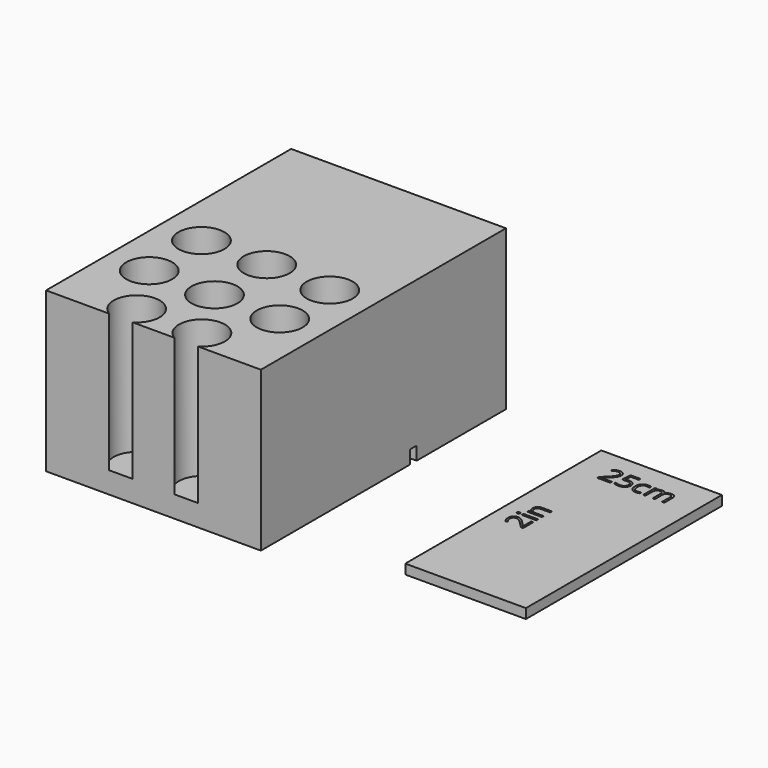
from build123d import *

# Parameters (mm, degrees)
F0_W     = 44.5262
F0_H     = 63.5
F1_DEPTH = 33.02
F2_W     = 44.5262
F2_H     = 1.778
F3_DEPTH = 2.7686
F4_R     = 4.7625
F5_DEPTH = 28.575
F6_W     = 25
F6_H     = 50.8
F6_W_2   = 3.0738876539
F6_H_2   = 0.4657949467
F7_DEPTH = 2


# Not quite as in the source:
# - a length typed as a fraction of an inch, garbled in the dataset ("3 / 203.2 mm" for 3/8 in), is restored


with BuildPart() as f1:
    # F0 (on Top) → F1 (new body)
    with BuildSketch(Plane.XY):
        Rectangle(F0_W, F0_H)
    extrude(amount=F1_DEPTH)

    # F2 (on face) → F3 (cut)
    with BuildSketch(Plane(origin=(0, 0, 0), x_dir=(1, 0, 0), z_dir=(0, 0, -1))):
        with Locations((0, -7.7216)):
            Rectangle(F2_W, F2_H)
    extrude(amount=-F3_DEPTH, mode=Mode.SUBTRACT)

    # F4 (on face) → F5 (cut)
    with BuildSketch(Plane.XY.offset(33.02)):
        with Locations((0, -15.9420263954)):
            Circle(F4_R)
        with Locations((-13.525, -15.9420263954)):
            Circle(F4_R)
        with Locations((13.525, -15.9420263954)):
            Circle(F4_R)
        with Locations((-6.7625, -27.6550199815)):
            Circle(F4_R)
        with Locations((6.7625, -27.6550199815)):
            Circle(F4_R)
        with Locations((0, -2.4170263954)):
            Circle(F4_R)
        with Locations((-13.525, -2.4170263954)):
            Circle(F4_R)
        with Locations((13.525, -2.9795283917)):
            Circle(F4_R)
    extrude(amount=-F5_DEPTH, mode=Mode.SUBTRACT)


with BuildPart() as f7:
    # F6 (on Top) → F7 (new body)
    with BuildSketch(Plane.XY):
        with Locations((58.2457509378, 1.7099808902)):
            Rectangle(F6_W, F6_H)
        with BuildLine():
            add(Edge.make_bspline(
                [(49.195293276, 1.4402865135), (49.1181095276, 1.361756537), (48.9610495745, 1.361756537)],
                knots=[0, 0, 0, 1, 1, 1], degree=2))
            add(Edge.make_bspline(
                [(48.9610495745, 1.361756537), (48.801297165, 1.361756537), (48.726805873, 1.4402865135)],
                knots=[0, 0, 0, 1, 1, 1], degree=2))
            add(Edge.make_bspline(
                [(48.726805873, 1.4402865135), (48.6523145809, 1.5188164901), (48.6523145809, 1.637284569)],
                knots=[0, 0, 0, 1, 1, 1], degree=2))
            add(Edge.make_bspline(
                [(48.6523145809, 1.637284569), (48.6523145809, 1.7494702498), (48.7281521012, 1.8306926827)],
                knots=[0, 0, 0, 1, 1, 1], degree=2))
            add(Edge.make_bspline(
                [(48.7281521012, 1.8306926827), (48.8039896214, 1.9119151156), (48.9610495745, 1.9119151156)],
                knots=[0, 0, 0, 1, 1, 1], degree=2))
            add(Edge.make_bspline(
                [(48.9610495745, 1.9119151156), (49.1181095276, 1.9119151156), (49.195293276, 1.8306926827)],
                knots=[0, 0, 0, 1, 1, 1], degree=2))
            add(Edge.make_bspline(
                [(49.195293276, 1.8306926827), (49.2724770244, 1.7494702498), (49.2724770244, 1.637284569)],
                knots=[0, 0, 0, 1, 1, 1], degree=2))
            add(Edge.make_bspline(
                [(49.2724770244, 1.637284569), (49.2724770244, 1.5188164901), (49.195293276, 1.4402865135)],
                knots=[0, 0, 0, 1, 1, 1], degree=2))
        make_face(mode=Mode.SUBTRACT)
        with BuildLine():
            Line((52.4361132229, 0.599791393), (52.8678037226, 0.599791393))
            Line((52.8678037226, 0.599791393), (52.8678037226, -2.0953574025))
            Line((52.8678037226, -2.0953574025), (52.4666277281, -2.0953574025))
            Line((52.4666277281, -2.0953574025), (51.3815678234, -1.0156824105))
            add(Edge.make_bspline(
                [(51.3815678234, -1.0156824105), (50.8816684298, -0.522065415), (50.6685156363, -0.3650054619)],
                knots=[0, 0, 0, 1, 1, 1], degree=2))
            add(Edge.make_bspline(
                [(50.6685156363, -0.3650054619), (50.4553628427, -0.2079455088), (50.2534286173, -0.1294155322)],
                knots=[0, 0, 0, 1, 1, 1], degree=2))
            add(Edge.make_bspline(
                [(50.2534286173, -0.1294155322), (50.0514943919, -0.0508855557), (49.8190456612, -0.0508855557)],
                knots=[0, 0, 0, 1, 1, 1], degree=2))
            add(Edge.make_bspline(
                [(49.8190456612, -0.0508855557), (49.4905659879, -0.0508855557), (49.2985041023, -0.2501273248)],
                knots=[0, 0, 0, 1, 1, 1], degree=2))
            add(Edge.make_bspline(
                [(49.2985041023, -0.2501273248), (49.1064422168, -0.4493690938), (49.1064422168, -0.8029783597)],
                knots=[0, 0, 0, 1, 1, 1], degree=2))
            add(Edge.make_bspline(
                [(49.1064422168, -0.8029783597), (49.1064422168, -1.0578642265), (49.1908058488, -1.2867230153)],
                knots=[0, 0, 0, 1, 1, 1], degree=2))
            add(Edge.make_bspline(
                [(49.1908058488, -1.2867230153), (49.2751694807, -1.5155818042), (49.496848386, -1.7955972634)],
                knots=[0, 0, 0, 1, 1, 1], degree=2))
            Line((49.496848386, -1.7955972634), (49.1800360234, -2.0424057612))
            add(Edge.make_bspline(
                [(49.1800360234, -2.0424057612), (48.7088561641, -1.4760924445), (48.7088561641, -0.8083632724)],
                knots=[0, 0, 0, 1, 1, 1], degree=2))
            add(Edge.make_bspline(
                [(48.7088561641, -0.8083632724), (48.7088561641, -0.2303826449), (49.0045776187, 0.0976482857)],
                knots=[0, 0, 0, 1, 1, 1], degree=2))
            add(Edge.make_bspline(
                [(49.0045776187, 0.0976482857), (49.3002990732, 0.4256792164), (49.7993009814, 0.4256792164)],
                knots=[0, 0, 0, 1, 1, 1], degree=2))
            add(Edge.make_bspline(
                [(49.7993009814, 0.4256792164), (50.1897071506, 0.4256792164), (50.5711384653, 0.2066927675)],
                knots=[0, 0, 0, 1, 1, 1], degree=2))
            add(Edge.make_bspline(
                [(50.5711384653, 0.2066927675), (50.95256978, -0.0122936815), (51.5359353202, -0.6118139596)],
                knots=[0, 0, 0, 1, 1, 1], degree=2))
            Line((51.5359353202, -0.6118139596), (52.4136760867, -1.509299406))
            Line((52.4136760867, -1.509299406), (52.4361132229, -1.509299406))
            Line((52.4361132229, -1.509299406), (52.4361132229, 0.599791393))
        make_face(mode=Mode.SUBTRACT)
        with Locations((51.3308598957, 1.6341433699)):
            Rectangle(F6_W_2, F6_H_2, mode=Mode.SUBTRACT)
        with BuildLine():
            Line((52.8678037226, 5.4237756673), (52.8678037226, 4.9579807206))
            Line((52.8678037226, 4.9579807206), (50.8789759734, 4.9579807206))
            add(Edge.make_bspline(
                [(50.8789759734, 4.9579807206), (50.5038270568, 4.9579807206), (50.3184963122, 4.7870097431)],
                knots=[0, 0, 0, 1, 1, 1], degree=2))
            add(Edge.make_bspline(
                [(50.3184963122, 4.7870097431), (50.1331655675, 4.6160387656), (50.1331655675, 4.2507621889)],
                knots=[0, 0, 0, 1, 1, 1], degree=2))
            add(Edge.make_bspline(
                [(50.1331655675, 4.2507621889), (50.1331655675, 3.7688125042), (50.3938850897, 3.5444411426)],
                knots=[0, 0, 0, 1, 1, 1], degree=2))
            add(Edge.make_bspline(
                [(50.3938850897, 3.5444411426), (50.6546046118, 3.320069781), (51.2550223755, 3.320069781)],
                knots=[0, 0, 0, 1, 1, 1], degree=2))
            Line((51.2550223755, 3.320069781), (52.8678037226, 3.320069781))
            Line((52.8678037226, 3.320069781), (52.8678037226, 2.8542748343))
            Line((52.8678037226, 2.8542748343), (49.7939160687, 2.8542748343))
            Line((49.7939160687, 2.8542748343), (49.7939160687, 3.2330136927))
            Line((49.7939160687, 3.2330136927), (50.2148367431, 3.3084024702))
            Line((50.2148367431, 3.3084024702), (50.2148367431, 3.3308396063))
            add(Edge.make_bspline(
                [(50.2148367431, 3.3308396063), (49.9877729252, 3.4744372777), (49.8625737054, 3.7324643436)],
                knots=[0, 0, 0, 1, 1, 1], degree=2))
            add(Edge.make_bspline(
                [(49.8625737054, 3.7324643436), (49.7373744856, 3.9904914094), (49.7373744856, 4.307303772)],
                knots=[0, 0, 0, 1, 1, 1], degree=2))
            add(Edge.make_bspline(
                [(49.7373744856, 4.307303772), (49.7373744856, 4.8628472633), (50.0052738914, 5.1433114653)],
                knots=[0, 0, 0, 1, 1, 1], degree=2))
            add(Edge.make_bspline(
                [(50.0052738914, 5.1433114653), (50.2731732971, 5.4237756673), (50.8628212354, 5.4237756673)],
                knots=[0, 0, 0, 1, 1, 1], degree=2))
            Line((50.8628212354, 5.4237756673), (52.8678037226, 5.4237756673))
        make_face(mode=Mode.SUBTRACT)
        with BuildLine():
            Line((53.9458981642, 19.6119133069), (53.9458981642, 19.1802228072))
            Line((53.9458981642, 19.1802228072), (51.2507493687, 19.1802228072))
            Line((51.2507493687, 19.1802228072), (51.2507493687, 19.5813988017))
            Line((51.2507493687, 19.5813988017), (52.3304243607, 20.6664587064))
            add(Edge.make_bspline(
                [(52.3304243607, 20.6664587064), (52.8240413562, 21.1663581), (52.9811013093, 21.3795108936)],
                knots=[0, 0, 0, 1, 1, 1], degree=2))
            add(Edge.make_bspline(
                [(52.9811013093, 21.3795108936), (53.1381612624, 21.5926636871), (53.216691239, 21.7945979125)],
                knots=[0, 0, 0, 1, 1, 1], degree=2))
            add(Edge.make_bspline(
                [(53.216691239, 21.7945979125), (53.2952212156, 21.996532138), (53.2952212156, 22.2289808686)],
                knots=[0, 0, 0, 1, 1, 1], degree=2))
            add(Edge.make_bspline(
                [(53.2952212156, 22.2289808686), (53.2952212156, 22.5574605419), (53.0959794465, 22.7495224275)],
                knots=[0, 0, 0, 1, 1, 1], degree=2))
            add(Edge.make_bspline(
                [(53.0959794465, 22.7495224275), (52.8967376774, 22.941584313), (52.5431284115, 22.941584313)],
                knots=[0, 0, 0, 1, 1, 1], degree=2))
            add(Edge.make_bspline(
                [(52.5431284115, 22.941584313), (52.2882425447, 22.941584313), (52.0593837559, 22.857220681)],
                knots=[0, 0, 0, 1, 1, 1], degree=2))
            add(Edge.make_bspline(
                [(52.0593837559, 22.857220681), (51.8305249671, 22.7728570491), (51.5505095078, 22.5511781438)],
                knots=[0, 0, 0, 1, 1, 1], degree=2))
            Line((51.5505095078, 22.5511781438), (51.30370101, 22.8679905064))
            add(Edge.make_bspline(
                [(51.30370101, 22.8679905064), (51.8700143267, 23.3391703657), (52.5377434988, 23.3391703657)],
                knots=[0, 0, 0, 1, 1, 1], degree=2))
            add(Edge.make_bspline(
                [(52.5377434988, 23.3391703657), (53.1157241263, 23.3391703657), (53.4437550569, 23.0434489112)],
                knots=[0, 0, 0, 1, 1, 1], degree=2))
            add(Edge.make_bspline(
                [(53.4437550569, 23.0434489112), (53.7717859876, 22.7477274566), (53.7717859876, 22.2487255484)],
                knots=[0, 0, 0, 1, 1, 1], degree=2))
            add(Edge.make_bspline(
                [(53.7717859876, 22.2487255484), (53.7717859876, 21.8583193792), (53.5527995387, 21.4768880645)],
                knots=[0, 0, 0, 1, 1, 1], degree=2))
            add(Edge.make_bspline(
                [(53.5527995387, 21.4768880645), (53.3338130898, 21.0954567498), (52.7342928116, 20.5120912096)],
                knots=[0, 0, 0, 1, 1, 1], degree=2))
            Line((52.7342928116, 20.5120912096), (51.8368073652, 19.6343504431))
            Line((51.8368073652, 19.6343504431), (51.8368073652, 19.6119133069))
            Line((51.8368073652, 19.6119133069), (53.9458981642, 19.6119133069))
        make_face(mode=Mode.SUBTRACT)
        with BuildLine():
            add(Edge.make_bspline(
                [(55.1736582548, 21.6204857359), (55.4958555301, 21.6851046881), (55.8162578345, 21.6851046881)],
                knots=[0, 0, 0, 1, 1, 1], degree=2))
            add(Edge.make_bspline(
                [(55.8162578345, 21.6851046881), (56.4642423268, 21.6851046881), (56.8358013016, 21.3638048983)],
                knots=[0, 0, 0, 1, 1, 1], degree=2))
            add(Edge.make_bspline(
                [(56.8358013016, 21.3638048983), (57.2073602764, 21.0425051084), (57.2073602764, 20.4842691608)],
                knots=[0, 0, 0, 1, 1, 1], degree=2))
            add(Edge.make_bspline(
                [(57.2073602764, 20.4842691608), (57.2073602764, 19.8479519793), (56.8021455973, 19.4858166017)],
                knots=[0, 0, 0, 1, 1, 1], degree=2))
            add(Edge.make_bspline(
                [(56.8021455973, 19.4858166017), (56.3969309183, 19.1236812241), (55.6843274738, 19.1236812241)],
                knots=[0, 0, 0, 1, 1, 1], degree=2))
            add(Edge.make_bspline(
                [(55.6843274738, 19.1236812241), (54.9914687092, 19.1236812241), (54.627089618, 19.3453601293)],
                knots=[0, 0, 0, 1, 1, 1], degree=2))
            Line((54.627089618, 19.3453601293), (54.627089618, 19.7941028525))
            add(Edge.make_bspline(
                [(54.627089618, 19.7941028525), (54.8227414453, 19.66845489), (55.1144242154, 19.5966560543)],
                knots=[0, 0, 0, 1, 1, 1], degree=2))
            add(Edge.make_bspline(
                [(55.1144242154, 19.5966560543), (55.4061069855, 19.5248572186), (55.6897123865, 19.5248572186)],
                knots=[0, 0, 0, 1, 1, 1], degree=2))
            add(Edge.make_bspline(
                [(55.6897123865, 19.5248572186), (56.183329382, 19.5248572186), (56.4566137005, 19.7577546919)],
                knots=[0, 0, 0, 1, 1, 1], degree=2))
            add(Edge.make_bspline(
                [(56.4566137005, 19.7577546919), (56.7298980189, 19.9906521653), (56.7298980189, 20.4313175195)],
                knots=[0, 0, 0, 1, 1, 1], degree=2))
            add(Edge.make_bspline(
                [(56.7298980189, 20.4313175195), (56.7298980189, 21.2893136062), (55.6789425612, 21.2893136062)],
                knots=[0, 0, 0, 1, 1, 1], degree=2))
            add(Edge.make_bspline(
                [(55.6789425612, 21.2893136062), (55.4123893836, 21.2893136062), (54.9663391167, 21.2076424306)],
                knots=[0, 0, 0, 1, 1, 1], degree=2))
            Line((54.9663391167, 21.2076424306), (54.7249155317, 21.3620099274))
            Line((54.7249155317, 21.3620099274), (54.8792830284, 23.2808338117))
            Line((54.8792830284, 23.2808338117), (56.9183699626, 23.2808338117))
            Line((56.9183699626, 23.2808338117), (56.9183699626, 22.8518357684))
            Line((56.9183699626, 22.8518357684), (55.2777665666, 22.8518357684))
            Line((55.2777665666, 22.8518357684), (55.1736582548, 21.6204857359))
        make_face(mode=Mode.SUBTRACT)
        with BuildLine():
            add(Edge.make_bspline(
                [(60.0362344034, 19.284331119), (59.7283968953, 19.1236812241), (59.2599094922, 19.1236812241)],
                knots=[0, 0, 0, 1, 1, 1], degree=2))
            add(Edge.make_bspline(
                [(59.2599094922, 19.1236812241), (58.5921803201, 19.1236812241), (58.226006258, 19.5347295585)],
                knots=[0, 0, 0, 1, 1, 1], degree=2))
            add(Edge.make_bspline(
                [(58.226006258, 19.5347295585), (57.8598321959, 19.945777893), (57.8598321959, 20.697870697)],
                knots=[0, 0, 0, 1, 1, 1], degree=2))
            add(Edge.make_bspline(
                [(57.8598321959, 20.697870697), (57.8598321959, 21.4688106955), (58.2318399134, 21.8897313698)],
                knots=[0, 0, 0, 1, 1, 1], degree=2))
            add(Edge.make_bspline(
                [(58.2318399134, 21.8897313698), (58.6038476309, 22.3106520442), (59.2904239974, 22.3106520442)],
                knots=[0, 0, 0, 1, 1, 1], degree=2))
            add(Edge.make_bspline(
                [(59.2904239974, 22.3106520442), (59.5121029027, 22.3106520442), (59.7337818079, 22.2626365728)],
                knots=[0, 0, 0, 1, 1, 1], degree=2))
            add(Edge.make_bspline(
                [(59.7337818079, 22.2626365728), (59.9554607132, 22.2146211014), (60.0811086757, 22.1500021493)],
                knots=[0, 0, 0, 1, 1, 1], degree=2))
            Line((60.0811086757, 22.1500021493), (59.9384084897, 21.7551085529))
            add(Edge.make_bspline(
                [(59.9384084897, 21.7551085529), (59.7840409929, 21.8170350487), (59.6018514473, 21.8574218938)],
                knots=[0, 0, 0, 1, 1, 1], degree=2))
            add(Edge.make_bspline(
                [(59.6018514473, 21.8574218938), (59.4196619017, 21.8978087389), (59.2796541721, 21.8978087389)],
                knots=[0, 0, 0, 1, 1, 1], degree=2))
            add(Edge.make_bspline(
                [(59.2796541721, 21.8978087389), (58.342679366, 21.8978087389), (58.342679366, 20.7032556097)],
                knots=[0, 0, 0, 1, 1, 1], degree=2))
            add(Edge.make_bspline(
                [(58.342679366, 20.7032556097), (58.342679366, 20.136942293), (58.5710894121, 19.8340409549)],
                knots=[0, 0, 0, 1, 1, 1], degree=2))
            add(Edge.make_bspline(
                [(58.5710894121, 19.8340409549), (58.7994994582, 19.5311396167), (59.2482421814, 19.5311396167)],
                knots=[0, 0, 0, 1, 1, 1], degree=2))
            add(Edge.make_bspline(
                [(59.2482421814, 19.5311396167), (59.6323659525, 19.5311396167), (60.0362344034, 19.6962769389)],
                knots=[0, 0, 0, 1, 1, 1], degree=2))
            Line((60.0362344034, 19.6962769389), (60.0362344034, 19.284331119))
        make_face(mode=Mode.SUBTRACT)
        with BuildLine():
            Line((65.1492089914, 19.1802228072), (64.6843115302, 19.1802228072))
            Line((64.6843115302, 19.1802228072), (64.6843115302, 21.1798203817))
            add(Edge.make_bspline(
                [(64.6843115302, 21.1798203817), (64.6843115302, 21.5477894148), (64.5272515771, 21.7313251885)],
                knots=[0, 0, 0, 1, 1, 1], degree=2))
            add(Edge.make_bspline(
                [(64.5272515771, 21.7313251885), (64.370191624, 21.9148609623), (64.0390194942, 21.9148609623)],
                knots=[0, 0, 0, 1, 1, 1], degree=2))
            add(Edge.make_bspline(
                [(64.0390194942, 21.9148609623), (63.6046365382, 21.9148609623), (63.3968686574, 21.6653600082)],
                knots=[0, 0, 0, 1, 1, 1], degree=2))
            add(Edge.make_bspline(
                [(63.3968686574, 21.6653600082), (63.1891007765, 21.4158590541), (63.1891007765, 20.8971124661)],
                knots=[0, 0, 0, 1, 1, 1], degree=2))
            Line((63.1891007765, 20.8971124661), (63.1891007765, 19.1802228072))
            Line((63.1891007765, 19.1802228072), (62.7233058298, 19.1802228072))
            Line((62.7233058298, 19.1802228072), (62.7233058298, 21.1798203817))
            add(Edge.make_bspline(
                [(62.7233058298, 21.1798203817), (62.7233058298, 21.5477894148), (62.5662458767, 21.7313251885)],
                knots=[0, 0, 0, 1, 1, 1], degree=2))
            add(Edge.make_bspline(
                [(62.5662458767, 21.7313251885), (62.4091859236, 21.9148609623), (62.0753213376, 21.9148609623)],
                knots=[0, 0, 0, 1, 1, 1], degree=2))
            add(Edge.make_bspline(
                [(62.0753213376, 21.9148609623), (61.6382459252, 21.9148609623), (61.4349654716, 21.652795212)],
                knots=[0, 0, 0, 1, 1, 1], degree=2))
            add(Edge.make_bspline(
                [(61.4349654716, 21.652795212), (61.231685018, 21.3907294616), (61.231685018, 20.7930041544)],
                knots=[0, 0, 0, 1, 1, 1], degree=2))
            Line((61.231685018, 20.7930041544), (61.231685018, 19.1802228072))
            Line((61.231685018, 19.1802228072), (60.7658900713, 19.1802228072))
            Line((60.7658900713, 19.1802228072), (60.7658900713, 22.2541104611))
            Line((60.7658900713, 22.2541104611), (61.1446289297, 22.2541104611))
            Line((61.1446289297, 22.2541104611), (61.2200177071, 21.8331897867))
            Line((61.2200177071, 21.8331897867), (61.2424548433, 21.8331897867))
            add(Edge.make_bspline(
                [(61.2424548433, 21.8331897867), (61.3743852039, 22.0575611483), (61.6144625608, 22.1841065963)],
                knots=[0, 0, 0, 1, 1, 1], degree=2))
            add(Edge.make_bspline(
                [(61.6144625608, 22.1841065963), (61.8545399177, 22.3106520442), (62.1516076005, 22.3106520442)],
                knots=[0, 0, 0, 1, 1, 1], degree=2))
            add(Edge.make_bspline(
                [(62.1516076005, 22.3106520442), (62.8722884139, 22.3106520442), (63.0939673192, 21.7883155144)],
                knots=[0, 0, 0, 1, 1, 1], degree=2))
            Line((63.0939673192, 21.7883155144), (63.1164044554, 21.7883155144))
            add(Edge.make_bspline(
                [(63.1164044554, 21.7883155144), (63.2537197287, 22.0297390995), (63.5144392508, 22.1701955718)],
                knots=[0, 0, 0, 1, 1, 1], degree=2))
            add(Edge.make_bspline(
                [(63.5144392508, 22.1701955718), (63.775158773, 22.3106520442), (64.1090233591, 22.3106520442)],
                knots=[0, 0, 0, 1, 1, 1], degree=2))
            add(Edge.make_bspline(
                [(64.1090233591, 22.3106520442), (64.6304624034, 22.3106520442), (64.8898356974, 22.0427526384)],
                knots=[0, 0, 0, 1, 1, 1], degree=2))
            add(Edge.make_bspline(
                [(64.8898356974, 22.0427526384), (65.1492089914, 21.7748532327), (65.1492089914, 21.1852052944)],
                knots=[0, 0, 0, 1, 1, 1], degree=2))
            Line((65.1492089914, 21.1852052944), (65.1492089914, 19.1802228072))
        make_face(mode=Mode.SUBTRACT)
    extrude(amount=F7_DEPTH)


solid = Compound([f1.part, f7.part])
